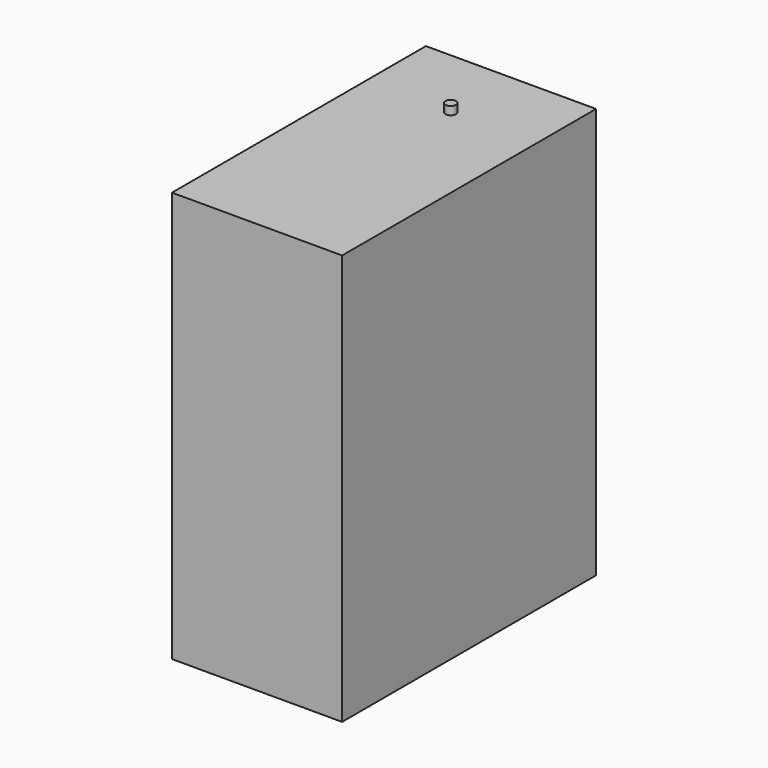
from build123d import *

# Parameters (mm, degrees)
F0_W     = 520
F0_H     = 970
F1_DEPTH = 1255
F2_R     = 80
F3_DEPTH = 50
F5_R     = 7.5
F6_DEPTH = 20
F7_R     = 16
F8_DEPTH = 25


# Not quite as in the source:
# - the program builds the solid bodies; features that only make, move or delete a surface that nothing else refers to are left out


with BuildPart() as f1:
    # F0 (on Top) → F1 (new body)
    with BuildSketch(Plane.XY):
        Rectangle(F0_W, F0_H)
    extrude(amount=F1_DEPTH)

    # F2 (on face) → F3 (join)
    with BuildSketch(Plane(origin=(0, 485, 0), x_dir=(-1, 0, 0), z_dir=(0, 1, 0))):
        with Locations((0, 930)):
            Circle(F2_R)
    extrude(amount=F3_DEPTH)

    # F5 (on face) → F6 (join)
    with BuildSketch(Plane(origin=(0, 485, 0), x_dir=(-1, 0, 0), z_dir=(0, 1, 0))):
        with Locations((0, 52.045196724)):
            Circle(F5_R)
    extrude(amount=F6_DEPTH)

    # F7 (on face) → F8 (join)
    with BuildSketch(Plane.XY.offset(1255)):
        with Locations((0, 255)):
            Circle(F7_R)
    extrude(amount=F8_DEPTH)


solid = f1.part
